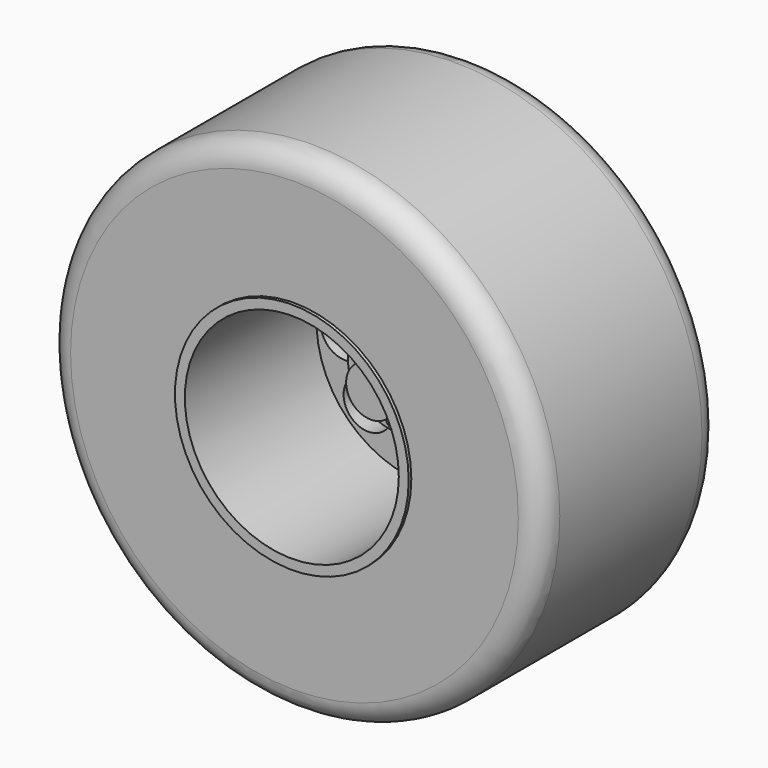
from build123d import *

# Parameters (mm, degrees)
F0_R      = 19.05
F1_DEPTH  = 17.272
F2_R      = 3.175
F3_DEPTH  = 10.16
F4_R      = 1.524
F5_DEPTH  = 9.398
F7_R      = 8.255
F8_DEPTH  = 12.446
F9_R      = 17.272
F9_R_2    = 8.89
F10_DEPTH = 15.24
F11_R     = 9.017
F11_R_2   = 8.255
F12_DEPTH = 0.254
F13_R     = 1.905
F14_DEPTH = 5.08
F15_R     = 3.81
F15_R_2   = 1.905
F16_DEPTH = 2.54
F17_R     = 1.905
F18_DEPTH = 14.987
F19_R     = 0.6985
F20_DEPTH = 0.254
F21_R     = 1.778
F22_R     = 1.77799


# Not quite as in the source:
# - a fillet or chamfer is up to 0.001 mm smaller than in the source, because OpenCascade refuses the exact size


with BuildPart() as f1:
    # F0 (on Front) → F1 (new body)
    with BuildSketch(Plane.XZ):
        Circle(F0_R)
    extrude(amount=F1_DEPTH)

    # F2 (on face) → F3 (join)
    with BuildSketch(Plane(origin=(0, 0, 0), x_dir=(-1, 0, 0), z_dir=(0, 1, 0))):
        Circle(F2_R)
    extrude(amount=F3_DEPTH)

    # F4 (on face) → F5 (cut)
    with BuildSketch(Plane(origin=(0, 10.16, 0), x_dir=(-1, 0, 0), z_dir=(0, 1, 0))):
        Circle(F4_R)
    extrude(amount=-F5_DEPTH, mode=Mode.SUBTRACT)

    # F7 (on face) → F8 (cut)
    with BuildSketch(Plane.XZ.offset(17.272)):
        Circle(F7_R)
    extrude(amount=-F8_DEPTH, mode=Mode.SUBTRACT)

    # F9 (on face) → F10 (cut)
    with BuildSketch(Plane(origin=(0, 0, 0), x_dir=(-1, 0, 0), z_dir=(0, 1, 0))):
        Circle(F9_R)
        Circle(F9_R_2, mode=Mode.SUBTRACT)
    extrude(amount=-F10_DEPTH, mode=Mode.SUBTRACT)

    # F11 (on face) → F12 (join)
    with BuildSketch(Plane.XZ.offset(17.272)):
        Circle(F11_R)
        Circle(F11_R_2, mode=Mode.SUBTRACT)
    extrude(amount=F12_DEPTH)

    # F13 (on face) → F14 (join)
    with BuildSketch(Plane.XZ.offset(4.826)):
        Circle(F13_R)
    extrude(amount=F14_DEPTH)

    # F15 (on face) → F16 (join)
    with BuildSketch(Plane.XZ.offset(4.826)):
        Circle(F15_R)
        Circle(F15_R_2, mode=Mode.SUBTRACT)
    extrude(amount=F16_DEPTH)

    # F17 (on face) → F18 (cut, through all)
    with BuildSketch(Plane.XZ.offset(4.826)):
        with Locations((-4.2682749969, 4.2629666667)):
            Circle(F17_R)
        with Locations((0, 6.0325)):
            Circle(F17_R)
        with Locations((4.2629666667, 4.2682749969)):
            Circle(F17_R)
        with Locations((6.0325, 0)):
            Circle(F17_R)
        with Locations((4.2682749969, -4.2629666667)):
            Circle(F17_R)
        with Locations((0, -6.0325)):
            Circle(F17_R)
        with Locations((-4.2629666667, -4.2682749969)):
            Circle(F17_R)
        with Locations((-6.0325, 0)):
            Circle(F17_R)
    extrude(amount=-F18_DEPTH, mode=Mode.SUBTRACT)

    # F19 (on face) → F20 (join)
    with BuildSketch(Plane.XZ.offset(7.366)):
        with Locations((-1.6795963584, 2.3117660614)):
            Circle(F19_R)
        with Locations((0, 2.8575)):
            Circle(F19_R)
        with Locations((1.6795963584, 2.3117660614)):
            Circle(F19_R)
        with Locations((2.7176439953, 0.8830160614)):
            Circle(F19_R)
        with Locations((1.6795963584, -2.3117660614)):
            Circle(F19_R)
        with Locations((0, -2.8575)):
            Circle(F19_R)
        with Locations((2.7176439953, -0.8830160614)):
            Circle(F19_R)
        with Locations((-1.6795963584, -2.3117660614)):
            Circle(F19_R)
        with Locations((-2.7176439953, -0.8830160614)):
            Circle(F19_R)
        with Locations((-2.7176439953, 0.8830160614)):
            Circle(F19_R)
    extrude(amount=F20_DEPTH)

    # F21
    f21_edges = [f1.edges().sort_by_distance(p)[0] for p in [
        (-19.05, -17.272, 0),
    ]]
    fillet(f21_edges, radius=F21_R)

    # F22 (radius 1.778 in the source; OpenCascade refuses exactly that, so slightly less here)
    f22_edges = [f1.edges().sort_by_distance(p)[0] for p in [
        (-19.05, 0, 0),
    ]]
    fillet(f22_edges, radius=F22_R)


solid = f1.part
